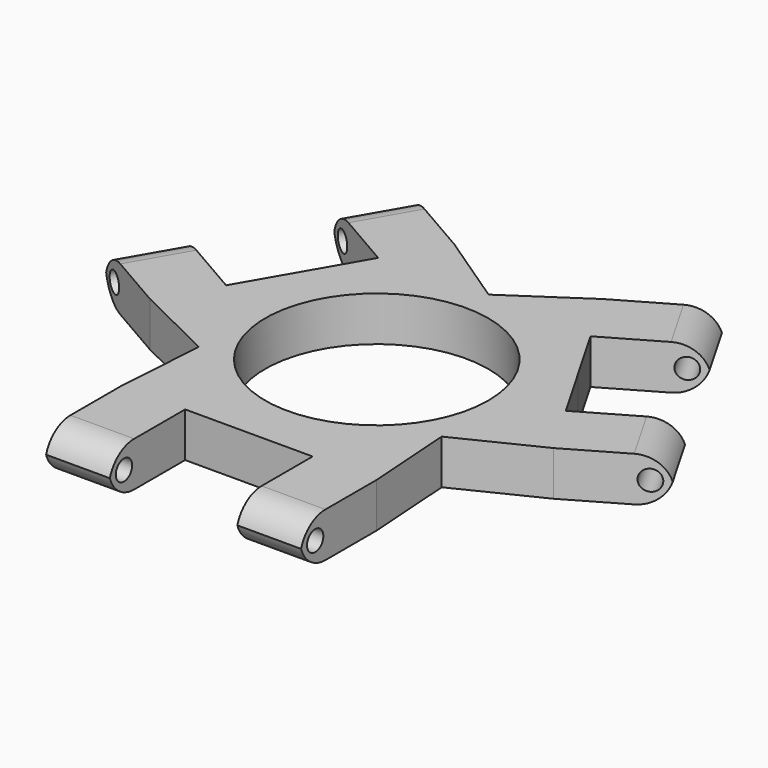
from build123d import *

# Parameters (mm, degrees)
F0_W          = 10
F0_H          = 15
F1_DEPTH      = 7
F3_DEPTH      = 60
F4_R          = 1.6
F5_DEPTH      = 60
F6_R          = 1.6
F7_DEPTH      = 60
F8_R          = 17.5
F9_DEPTH      = 25
F10_T1_DEPTH  = 35
F10_T3_DEPTH  = 35
F10_T5_DEPTH  = 35
F10_T7_DEPTH  = 35
F10_T9_DEPTH  = 35
F10_T11_DEPTH = 35


# Not quite as in the source:
# - a fillet or chamfer that OpenCascade refuses, or shapes differently, is made with other operations: its cross-section is extruded or revolved along the edge and cut away or added
# - a feature names something its author has since deleted; it is built from what else it names


with BuildPart() as f1:
    # F0 (on Top) → F1 (new body)
    with BuildSketch(Plane.XY):
        Polygon((-19.0935776077, -11.020506829), (-0.0410187244, -0.020506829), (-21.6916538191, 12.479493171), (-26.6916538191, 3.8192391331), (-31.6916538191, -4.8410149047), align=None)
        Polygon((-0.0410187244, 21.979493171), (-0.0410187244, -0.020506829), (21.6096163702, 12.479493171), (16.6096163702, 21.1397472088), (11.6096163702, 29.8000012467), align=None)
        Polygon((19.0115401588, -11.020506829), (-0.0410187244, -0.020506829), (-0.0410187244, -25.020506829), (9.9589812756, -25.020506829), (19.9589812756, -25.020506829), align=None)
        Polygon((-0.0410187244, -25.020506829), (-0.0410187244, -0.020506829), (-19.0935776077, -11.020506829), (-20.0410187244, -25.020506829), (-10.0410187244, -25.020506829), align=None)
        Polygon((-21.6916538191, 12.479493171), (-0.0410187244, -0.020506829), (-0.0410187244, 21.979493171), (-11.6916538191, 29.8000012467), (-16.6916538191, 21.1397472088), align=None)
        Polygon((21.6096163702, 12.479493171), (-0.0410187244, -0.020506829), (19.0115401588, -11.020506829), (31.6096163702, -4.8410149047), (26.6096163702, 3.8192391331), align=None)
        Polygon((-29.6820348758, 28.6397472088), (-16.6916538191, 21.1397472088), (-11.6916538191, 29.8000012467), (-24.6820348758, 37.3000012467), align=None)
        Polygon((-31.6916538191, -4.8410149047), (-26.6916538191, 3.8192391331), (-39.6820348758, 11.3192391331), (-44.6820348758, 2.6589850953), align=None)
        Polygon((39.5999974269, 11.3192391331), (26.6096163702, 3.8192391331), (31.6096163702, -4.8410149047), (44.5999974269, 2.6589850953), align=None)
        Polygon((11.6096163702, 29.8000012467), (16.6096163702, 21.1397472088), (29.5999974269, 28.6397472088), (24.5999974269, 37.3000012467), align=None)
        with Locations((-15.0410187244, -32.520506829)):
            Rectangle(F0_W, F0_H)
        with Locations((14.9589812756, -32.520506829)):
            Rectangle(F0_W, F0_H)
    extrude(amount=F1_DEPTH)

    # F2 (on face) → F3 (cut)
    with BuildSketch(Plane.YZ.offset(19.9589812756)):
        with BuildLine():
            ThreePointArc((-35.420506829, 3.5), (-37.020506829, 5.1), (-38.620506829, 3.5))
            ThreePointArc((-38.620506829, 3.5), (-37.020506829, 1.9), (-35.420506829, 3.5))
        make_face()
    extrude(amount=-F3_DEPTH, mode=Mode.SUBTRACT)

    # F4 (on face) → F5 (cut)
    with BuildSketch(Plane(origin=(9.9986250363, -17.3181265688, 0), x_dir=(0.8660254038, 0.5, 0), z_dir=(0.5, -0.8660254038, 0))):
        with Locations((36.9542233281, 3.5)):
            Circle(F4_R)
    extrude(amount=-F5_DEPTH, mode=Mode.SUBTRACT)

    # F6 (on face) → F7 (cut)
    with BuildSketch(Plane(origin=(9.9808656014, 17.2873663252, 0), x_dir=(-0.8660254038, 0.5, 0), z_dir=(0.5, 0.8660254038, 0))):
        with Locations((37.0252698429, 3.5)):
            Circle(F6_R)
    extrude(amount=-F7_DEPTH, mode=Mode.SUBTRACT)

    # F8 (on face) → F9 (cut)
    with BuildSketch(Plane.XY.offset(7)):
        Circle(F8_R)
    extrude(amount=-F9_DEPTH, mode=Mode.SUBTRACT)

    # F10: fillet of radius 5 on 12 edges, made by hand

    # F10_s2 → F10_t1 (cut)
    with BuildSketch(Plane.YZ.offset(-32.5410187244)):
        with BuildLine():
            ThreePointArc((-35.020506829, 7), (-38.556040735, 5.5355339059), (-40.020506829, 2))
            Line((-40.020506829, 2), (-40.020506829, 7))
            Line((-40.020506829, 7), (-35.020506829, 7))
        make_face()
        with BuildLine():
            ThreePointArc((-35.020506829, 0), (-38.556040735, 1.4644660941), (-40.020506829, 5))
            Line((-40.020506829, 5), (-40.020506829, 0))
            Line((-40.020506829, 0), (-35.020506829, 0))
        make_face()
    extrude(amount=F10_T1_DEPTH, mode=Mode.SUBTRACT)

    # F10_s4 → F10_t3 (cut)
    with BuildSketch(Plane.YZ.offset(-2.5410187244)):
        with BuildLine():
            ThreePointArc((-35.020506829, 0), (-38.556040735, 1.4644660941), (-40.020506829, 5))
            Line((-40.020506829, 5), (-40.020506829, 0))
            Line((-40.020506829, 0), (-35.020506829, 0))
        make_face()
        with BuildLine():
            ThreePointArc((-35.020506829, 7), (-38.556040735, 5.5355339059), (-40.020506829, 2))
            Line((-40.020506829, 2), (-40.020506829, 7))
            Line((-40.020506829, 7), (-35.020506829, 7))
        make_face()
    extrude(amount=F10_T3_DEPTH, mode=Mode.SUBTRACT)

    # F10_s6 → F10_t5 (cut)
    with BuildSketch(Plane(origin=(16.2486250363, -28.1434441161, 0), x_dir=(0, 0, 1), z_dir=(-0.5, 0.8660254038, 0))):
        with BuildLine():
            ThreePointArc((7, 34.9542233281), (5.5355339059, 38.489757234), (2, 39.9542233281))
            Line((2, 39.9542233281), (7, 39.9542233281))
            Line((7, 39.9542233281), (7, 34.9542233281))
        make_face()
        with BuildLine():
            ThreePointArc((0, 34.9542233281), (1.4644660941, 38.489757234), (5, 39.9542233281))
            Line((5, 39.9542233281), (0, 39.9542233281))
            Line((0, 39.9542233281), (0, 34.9542233281))
        make_face()
    extrude(amount=F10_T5_DEPTH, mode=Mode.SUBTRACT)

    # F10_s8 → F10_t7 (cut)
    with BuildSketch(Plane(origin=(1.2486250363, -2.1626820025, 0), x_dir=(0, 0, 1), z_dir=(-0.5, 0.8660254038, 0))):
        with BuildLine():
            ThreePointArc((7, 34.9542233281), (5.5355339059, 38.489757234), (2, 39.9542233281))
            Line((2, 39.9542233281), (7, 39.9542233281))
            Line((7, 39.9542233281), (7, 34.9542233281))
        make_face()
        with BuildLine():
            ThreePointArc((0, 34.9542233281), (1.4644660941, 38.489757234), (5, 39.9542233281))
            Line((5, 39.9542233281), (0, 39.9542233281))
            Line((0, 39.9542233281), (0, 34.9542233281))
        make_face()
    extrude(amount=F10_T7_DEPTH, mode=Mode.SUBTRACT)

    # F10_s10 → F10_t9 (cut)
    with BuildSketch(Plane(origin=(16.2308656014, 28.1126838725, 0), x_dir=(0, 0, 1), z_dir=(-0.5, -0.8660254038, 0))):
        with BuildLine():
            ThreePointArc((7, 35.0252698429), (5.5355339059, 38.5608037488), (2, 40.0252698429))
            Line((2, 40.0252698429), (7, 40.0252698429))
            Line((7, 40.0252698429), (7, 35.0252698429))
        make_face()
        with BuildLine():
            ThreePointArc((0, 35.0252698429), (1.4644660941, 38.5608037488), (5, 40.0252698429))
            Line((5, 40.0252698429), (0, 40.0252698429))
            Line((0, 40.0252698429), (0, 35.0252698429))
        make_face()
    extrude(amount=F10_T9_DEPTH, mode=Mode.SUBTRACT)

    # F10_s12 → F10_t11 (cut)
    with BuildSketch(Plane(origin=(1.2308656014, 2.131921759, 0), x_dir=(0, 0, 1), z_dir=(-0.5, -0.8660254038, 0))):
        with BuildLine():
            ThreePointArc((7, 35.0252698429), (5.5355339059, 38.5608037488), (2, 40.0252698429))
            Line((2, 40.0252698429), (7, 40.0252698429))
            Line((7, 40.0252698429), (7, 35.0252698429))
        make_face()
        with BuildLine():
            ThreePointArc((0, 35.0252698429), (1.4644660941, 38.5608037488), (5, 40.0252698429))
            Line((5, 40.0252698429), (0, 40.0252698429))
            Line((0, 40.0252698429), (0, 35.0252698429))
        make_face()
    extrude(amount=F10_T11_DEPTH, mode=Mode.SUBTRACT)


solid = f1.part
